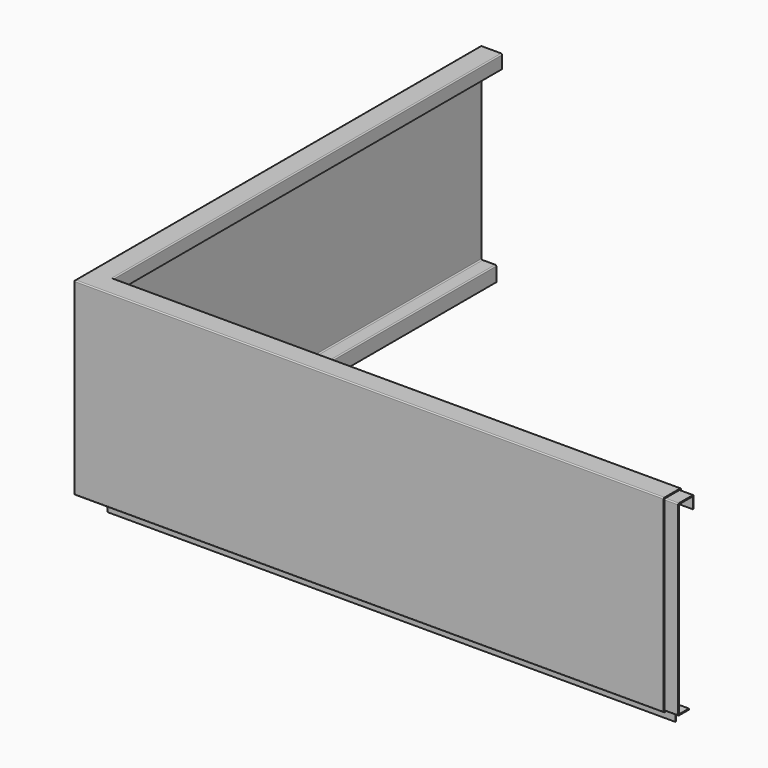
from build123d import *

# Parameters (mm, degrees)
F1_DEPTH       = 1051
F1_DEPTH_BACK  = 0.5
F3_DEPTH       = 900
F4_W           = 40
F4_H           = 40
F5_DEPTH       = 2
F7_DEPTH       = 346
F9_DEPTH       = 2
F14_D          = 5
F14_ON_F12_D   = 5
F16_DEPTH      = 25
F16_DEPTH_BACK = 25
F17_T1_DEPTH   = 50
F17_T3_DEPTH   = 1051.5
F17_T5_DEPTH   = 900
F17_T7_DEPTH   = 1069.0024143135
F17_T9_DEPTH   = 938
F17_T11_DEPTH  = 1031.5024143135
F17_T16_DEPTH  = 943.0024143135
F17_T21_DEPTH  = 1074.004828627
F17_T23_DEPTH  = 1056.0024143135
F17_T25_DEPTH  = 30.0024143135
F17_T27_DEPTH  = 1101.004828627
F17_T29_DEPTH  = 950.004828627
F17_T31_DEPTH  = 905.0024143135
F17_T33_DEPTH  = 910.004828627
F17_T38_DEPTH  = 1061.504828627
F17_T44_DEPTH  = 905.0024143135
F17_T49_DEPTH  = 1056.0024143135


# Not quite as in the source:
# - a fillet or chamfer that OpenCascade refuses, or shapes differently, is made with other operations: its cross-section is extruded or revolved along the edge and cut away or added


with BuildPart() as f1:
    # F0 (on Right) → F1 (new body, two sides)
    with BuildSketch(Plane.YZ) as f1_sk:
        Polygon((-40, 0), (-40, -350), (-13, -350), (-13, -376), (-11, -376), (-11, -348), (-38, -348), (-38, -2), (-2, -2), (-2, -25), (0, -25), (0, 0), align=None)
    extrude(amount=F1_DEPTH)
    extrude(f1_sk.sketch, amount=-F1_DEPTH_BACK)

    # F2 (on Front) → F3 (join)
    with BuildSketch(Plane.XZ):
        Polygon((-40, 0), (-40, -350), (-13, -350), (-13, -376), (-11, -376), (-11, -348), (-38, -348), (-38, -2), (-2, -2), (-2, -25), (0, -25), (0, 0), align=None)
    extrude(amount=-F3_DEPTH)

    # F4 (on Top) → F5 (join)
    with BuildSketch(Plane.XY):
        with Locations((-20, -20)):
            Rectangle(F4_W, F4_H)
    extrude(amount=-F5_DEPTH)

    # F6 (on face) → F7 (join)
    with BuildSketch(Plane(origin=(0, 0, -2), x_dir=(1, 0, 0), z_dir=(0, 0, -1))):
        Polygon((-40, 40), (-40, 0), (-38, 0), (-38, 38), (-0.5, 38), (-0.5, 40), align=None)
    extrude(amount=F7_DEPTH)

    # F8 (on face) → F9 (join)
    with BuildSketch(Plane(origin=(0, 0, -348), x_dir=(1, 0, 0), z_dir=(0, 0, -1))):
        Polygon((-40, 40), (-40, 0), (-11, 0), (-38, 38), (-0.5, 11), (0, 40), align=None)
    extrude(amount=F9_DEPTH)

    # F10: union 

    # F11: union 

    # F14 (through all)
    with Locations(Plane(origin=(-13, 0, 0), x_dir=(0, -1, 0), z_dir=(-1, 0, 0))):
        with Locations((-450, -363)):
            Hole(F14_D / 2)

    # F14 on F12 (through all)
    with Locations(Plane.XZ.offset(13)):
        with Locations((525.25, -363)):
            Hole(F14_ON_F12_D / 2)

    # F15 (on face) → F16 (join, two sides)
    with BuildSketch(Plane.YZ.offset(1051)) as f16_sk:
        Polygon((-13, -346), (-36, -346), (-36, -4), (-4, -4), (-4, -25), (-2, -25), (-2, -2), (-38, -2), (-38, -348), (-13, -348), align=None)
    extrude(amount=F16_DEPTH)
    extrude(f16_sk.sketch, amount=-F16_DEPTH_BACK)

    # F17: fillet of radius 2 on 21 edges, made by hand

    # F17_s2 → F17_t1 (join)
    with BuildSketch(Plane.YZ.offset(1026)):
        with BuildLine():
            ThreePointArc((-33.9990343146, -346.0004), (-35.4142135624, -345.4142135624), (-36.0004, -343.9990343146))
            Line((-36.0004, -343.9990343146), (-36.2005365685, -343.9990343146))
            ThreePointArc((-36.2005365685, -343.9990343146), (-36.2001365685, -344.9995171573), (-36.2001365685, -346))
            Line((-36.2001365685, -346), (-36, -346.2001365685))
            ThreePointArc((-36, -346.2001365685), (-34.9995171573, -346.2001365685), (-33.9990343146, -346.2005365685))
            Line((-33.9990343146, -346.2005365685), (-33.9990343146, -346.0004))
        make_face()
        with BuildLine():
            ThreePointArc((-6.0009656854, -3.9996), (-4.5857864376, -4.5857864376), (-3.9996, -6.0009656854))
            Line((-3.9996, -6.0009656854), (-3.7994634315, -6.0009656854))
            ThreePointArc((-3.7994634315, -6.0009656854), (-3.7998634315, -5.0004828427), (-3.7998634315, -4))
            Line((-3.7998634315, -4), (-4, -3.7998634315))
            ThreePointArc((-4, -3.7998634315), (-5.0004828427, -3.7998634315), (-6.0009656854, -3.7994634315))
            Line((-6.0009656854, -3.7994634315), (-6.0009656854, -3.9996))
        make_face()
    extrude(amount=F17_T1_DEPTH)

    # F17_s4 → F17_t3 (join)
    with BuildSketch(Plane.YZ.offset(-0.5)):
        with BuildLine():
            ThreePointArc((-15.0009656854, -349.9996), (-13.5857864376, -350.5857864376), (-12.9996, -352.0009656854))
            Line((-12.9996, -352.0009656854), (-12.7994634315, -352.0009656854))
            ThreePointArc((-12.7994634315, -352.0009656854), (-12.7998634315, -351.0004828427), (-12.7998634315, -350))
            Line((-12.7998634315, -350), (-13, -349.7998634315))
            ThreePointArc((-13, -349.7998634315), (-14.0004828427, -349.7998634315), (-15.0009656854, -349.7994634315))
            Line((-15.0009656854, -349.7994634315), (-15.0009656854, -349.9996))
        make_face()
    extrude(amount=F17_T3_DEPTH)

    # F17_s6 → F17_t5 (join)
    with BuildSketch(Plane.XZ.offset(-900)):
        with BuildLine():
            ThreePointArc((-15.0009656854, -349.9996), (-13.5857864376, -350.5857864376), (-12.9996, -352.0009656854))
            Line((-12.9996, -352.0009656854), (-12.7994634315, -352.0009656854))
            ThreePointArc((-12.7994634315, -352.0009656854), (-12.7998634315, -351.0004828427), (-12.7998634315, -350))
            Line((-12.7998634315, -350), (-13, -349.7998634315))
            ThreePointArc((-13, -349.7998634315), (-14.0004828427, -349.7998634315), (-15.0009656854, -349.7994634315))
            Line((-15.0009656854, -349.7994634315), (-15.0009656854, -349.9996))
        make_face()
        with BuildLine():
            ThreePointArc((-4.0009656854, -1.9996), (-2.5857864376, -2.5857864376), (-1.9996, -4.0009656854))
            Line((-1.9996, -4.0009656854), (-1.7994634315, -4.0009656854))
            ThreePointArc((-1.7994634315, -4.0009656854), (-1.7998634315, -3.0004828427), (-1.7998634315, -2))
            Line((-1.7998634315, -2), (-2, -1.7998634315))
            ThreePointArc((-2, -1.7998634315), (-3.0004828427, -1.7998634315), (-4.0009656854, -1.7994634315))
            Line((-4.0009656854, -1.7994634315), (-4.0009656854, -1.9996))
        make_face()
    extrude(amount=F17_T5_DEPTH)

    # F17_s8 → F17_t7 (join)
    with BuildSketch(Plane.YZ.offset(-38)):
        with BuildLine():
            ThreePointArc((-35.9990343146, -1.9996), (-37.4142135624, -2.5857864376), (-38.0004, -4.0009656854))
            Line((-38.0004, -4.0009656854), (-38.2005365685, -4.0009656854))
            ThreePointArc((-38.2005365685, -4.0009656854), (-38.2001365685, -3.0004828427), (-38.2001365685, -2))
            Line((-38.2001365685, -2), (-38, -1.7998634315))
            ThreePointArc((-38, -1.7998634315), (-36.9995171573, -1.7998634315), (-35.9990343146, -1.7994634315))
            Line((-35.9990343146, -1.7994634315), (-35.9990343146, -1.9996))
        make_face()
    extrude(amount=F17_T7_DEPTH)

    # F17_s10 → F17_t9 (join)
    with BuildSketch(Plane.XZ.offset(-900)):
        with BuildLine():
            ThreePointArc((-38.0004, -4.0009656854), (-37.4142135624, -2.5857864376), (-35.9990343146, -1.9996))
            Line((-35.9990343146, -1.9996), (-35.9990343146, -1.7994634315))
            ThreePointArc((-35.9990343146, -1.7994634315), (-36.9995171573, -1.7998634315), (-38, -1.7998634315))
            Line((-38, -1.7998634315), (-38.2001365685, -2))
            ThreePointArc((-38.2001365685, -2), (-38.2001365685, -3.0004828427), (-38.2005365685, -4.0009656854))
            Line((-38.2005365685, -4.0009656854), (-38.0004, -4.0009656854))
        make_face()
    extrude(amount=F17_T9_DEPTH)

    # F17_s12 → F17_t11 (join)
    with BuildSketch(Plane.YZ.offset(-0.5)):
        with BuildLine():
            ThreePointArc((-4.0009656854, -1.9996), (-2.5857864376, -2.5857864376), (-1.9996, -4.0009656854))
            Line((-1.9996, -4.0009656854), (-1.7994634315, -4.0009656854))
            ThreePointArc((-1.7994634315, -4.0009656854), (-1.7998634315, -3.0004828427), (-1.7998634315, -2))
            Line((-1.7998634315, -2), (-2, -1.7998634315))
            ThreePointArc((-2, -1.7998634315), (-3.0004828427, -1.7998634315), (-4.0009656854, -1.7994634315))
            Line((-4.0009656854, -1.7994634315), (-4.0009656854, -1.9996))
        make_face()
    extrude(amount=F17_T11_DEPTH)


with BuildPart() as f17_tool14:
    # F17_s15 → F17_t16 (new body)
    with BuildSketch(Plane.XZ.offset(-900)):
        with BuildLine():
            ThreePointArc((-35.9990343146, -348.0004), (-37.4142135624, -347.4142135624), (-38.0004, -345.9990343146))
            Line((-38.0004, -345.9990343146), (-38.2005365685, -345.9990343146))
            ThreePointArc((-38.2005365685, -345.9990343146), (-38.2001365685, -346.9995171573), (-38.2001365685, -348))
            Line((-38.2001365685, -348), (-38, -348.2001365685))
            ThreePointArc((-38, -348.2001365685), (-36.9995171573, -348.2001365685), (-35.9990343146, -348.2005365685))
            Line((-35.9990343146, -348.2005365685), (-35.9990343146, -348.0004))
        make_face()
    extrude(amount=F17_T16_DEPTH)

    split(bisect_by=Plane(origin=(-7.3097100782, 5.1937413714, 0), x_dir=(0, 0, 1), z_dir=(-0.8151804083, 0.5792071322, 0)), keep=Keep.TOP)


with BuildPart() as f1_1:
    add(f1.part)

    # F17_t13: union F17_tool14
    add(f17_tool14.part)


with BuildPart() as f17_tool19:
    # F17_s20 → F17_t21 (new body)
    with BuildSketch(Plane.YZ.offset(-43.0024143135)):
        with BuildLine():
            ThreePointArc((-35.9990343146, -348.0004), (-37.4142135624, -347.4142135624), (-38.0004, -345.9990343146))
            Line((-38.0004, -345.9990343146), (-38.2005365685, -345.9990343146))
            ThreePointArc((-38.2005365685, -345.9990343146), (-38.2001365685, -346.9995171573), (-38.2001365685, -348))
            Line((-38.2001365685, -348), (-38, -348.2001365685))
            ThreePointArc((-38, -348.2001365685), (-36.9995171573, -348.2001365685), (-35.9990343146, -348.2005365685))
            Line((-35.9990343146, -348.2005365685), (-35.9990343146, -348.0004))
        make_face()
    extrude(amount=F17_T21_DEPTH)

    split(bisect_by=Plane(origin=(5.0453108535, -7.0073761855, 0), x_dir=(0, 0, 1), z_dir=(0.5843047258, -0.8115343415, 0)), keep=Keep.TOP)


with BuildPart() as f1_2:
    add(f1_1.part)

    # F17_t18: union F17_tool19
    add(f17_tool19.part)

    # F17_s24 → F17_t23 (cut)
    with BuildSketch(Plane.YZ):
        with BuildLine():
            ThreePointArc((0.0004, -2.0009656854), (-0.5857864376, -0.5857864376), (-2.0009656854, 0.0004))
            Line((-2.0009656854, 0.0004), (-2.0009656854, 0.2005365685))
            ThreePointArc((-2.0009656854, 0.2005365685), (-1.0004828427, 0.2001365685), (0, 0.2001365685))
            Line((0, 0.2001365685), (0.2001365685, 0))
            ThreePointArc((0.2001365685, 0), (0.2001365685, -1.0004828427), (0.2005365685, -2.0009656854))
            Line((0.2005365685, -2.0009656854), (0.0004, -2.0009656854))
        make_face()
    extrude(amount=F17_T23_DEPTH, mode=Mode.SUBTRACT)

    # F17_s26 → F17_t25 (cut)
    with BuildSketch(Plane.YZ.offset(1051)):
        with BuildLine():
            ThreePointArc((-1.9996, -4.0009656854), (-2.5857864376, -2.5857864376), (-4.0009656854, -1.9996))
            Line((-4.0009656854, -1.9996), (-4.0009656854, -1.7994634315))
            ThreePointArc((-4.0009656854, -1.7994634315), (-3.0004828427, -1.7998634315), (-2, -1.7998634315))
            Line((-2, -1.7998634315), (-1.7998634315, -2))
            ThreePointArc((-1.7998634315, -2), (-1.7998634315, -3.0004828427), (-1.7994634315, -4.0009656854))
            Line((-1.7994634315, -4.0009656854), (-1.9996, -4.0009656854))
        make_face()
        with BuildLine():
            ThreePointArc((-35.9990343146, -1.9996), (-37.4142135624, -2.5857864376), (-38.0004, -4.0009656854))
            Line((-38.0004, -4.0009656854), (-38.2005365685, -4.0009656854))
            ThreePointArc((-38.2005365685, -4.0009656854), (-38.2001365685, -3.0004828427), (-38.2001365685, -2))
            Line((-38.2001365685, -2), (-38, -1.7998634315))
            ThreePointArc((-38, -1.7998634315), (-36.9995171573, -1.7998634315), (-35.9990343146, -1.7994634315))
            Line((-35.9990343146, -1.7994634315), (-35.9990343146, -1.9996))
        make_face()
        with BuildLine():
            ThreePointArc((-38.0004, -345.9990343146), (-37.4142135624, -347.4142135624), (-35.9990343146, -348.0004))
            Line((-35.9990343146, -348.0004), (-35.9990343146, -348.2005365685))
            ThreePointArc((-35.9990343146, -348.2005365685), (-36.9995171573, -348.2001365685), (-38, -348.2001365685))
            Line((-38, -348.2001365685), (-38.2001365685, -348))
            ThreePointArc((-38.2001365685, -348), (-38.2001365685, -346.9995171573), (-38.2005365685, -345.9990343146))
            Line((-38.2005365685, -345.9990343146), (-38.0004, -345.9990343146))
        make_face()
    extrude(amount=F17_T25_DEPTH, mode=Mode.SUBTRACT)

    # F17_s28 → F17_t27 (cut)
    with BuildSketch(Plane.YZ.offset(-45.0024143135)):
        with BuildLine():
            ThreePointArc((-40.0004, -2.0009656854), (-39.4142135624, -0.5857864376), (-37.9990343146, 0.0004))
            Line((-37.9990343146, 0.0004), (-37.9990343146, 0.2005365685))
            ThreePointArc((-37.9990343146, 0.2005365685), (-38.9995171573, 0.2001365685), (-40, 0.2001365685))
            Line((-40, 0.2001365685), (-40.2001365685, 0))
            ThreePointArc((-40.2001365685, 0), (-40.2001365685, -1.0004828427), (-40.2005365685, -2.0009656854))
            Line((-40.2005365685, -2.0009656854), (-40.0004, -2.0009656854))
        make_face()
        with BuildLine():
            ThreePointArc((-40.0004, -347.9990343146), (-39.4142135624, -349.4142135624), (-37.9990343146, -350.0004))
            Line((-37.9990343146, -350.0004), (-37.9990343146, -350.2005365685))
            ThreePointArc((-37.9990343146, -350.2005365685), (-38.9995171573, -350.2001365685), (-40, -350.2001365685))
            Line((-40, -350.2001365685), (-40.2001365685, -350))
            ThreePointArc((-40.2001365685, -350), (-40.2001365685, -348.9995171573), (-40.2005365685, -347.9990343146))
            Line((-40.2005365685, -347.9990343146), (-40.0004, -347.9990343146))
        make_face()
    extrude(amount=F17_T27_DEPTH, mode=Mode.SUBTRACT)

    # F17_s30 → F17_t29 (cut)
    with BuildSketch(Plane.XZ.offset(-905.0024143135)):
        with BuildLine():
            ThreePointArc((-40.0004, -2.0009656854), (-39.4142135624, -0.5857864376), (-37.9990343146, 0.0004))
            Line((-37.9990343146, 0.0004), (-37.9990343146, 0.2005365685))
            ThreePointArc((-37.9990343146, 0.2005365685), (-38.9995171573, 0.2001365685), (-40, 0.2001365685))
            Line((-40, 0.2001365685), (-40.2001365685, 0))
            ThreePointArc((-40.2001365685, 0), (-40.2001365685, -1.0004828427), (-40.2005365685, -2.0009656854))
            Line((-40.2005365685, -2.0009656854), (-40.0004, -2.0009656854))
        make_face()
        with BuildLine():
            ThreePointArc((-40.0004, -347.9990343146), (-39.4142135624, -349.4142135624), (-37.9990343146, -350.0004))
            Line((-37.9990343146, -350.0004), (-37.9990343146, -350.2005365685))
            ThreePointArc((-37.9990343146, -350.2005365685), (-38.9995171573, -350.2001365685), (-40, -350.2001365685))
            Line((-40, -350.2001365685), (-40.2001365685, -350))
            ThreePointArc((-40.2001365685, -350), (-40.2001365685, -348.9995171573), (-40.2005365685, -347.9990343146))
            Line((-40.2005365685, -347.9990343146), (-40.0004, -347.9990343146))
        make_face()
    extrude(amount=F17_T29_DEPTH, mode=Mode.SUBTRACT)

    # F17_s32 → F17_t31 (cut)
    with BuildSketch(Plane.XZ.offset(-905.0024143135)):
        with BuildLine():
            ThreePointArc((0.0004, -2.0009656854), (-0.5857864376, -0.5857864376), (-2.0009656854, 0.0004))
            Line((-2.0009656854, 0.0004), (-2.0009656854, 0.2005365685))
            ThreePointArc((-2.0009656854, 0.2005365685), (-1.0004828427, 0.2001365685), (0, 0.2001365685))
            Line((0, 0.2001365685), (0.2001365685, 0))
            ThreePointArc((0.2001365685, 0), (0.2001365685, -1.0004828427), (0.2005365685, -2.0009656854))
            Line((0.2005365685, -2.0009656854), (0.0004, -2.0009656854))
        make_face()
    extrude(amount=F17_T31_DEPTH, mode=Mode.SUBTRACT)

    # F17_s34 → F17_t33 (cut)
    with BuildSketch(Plane.XZ.offset(-905.0024143135)):
        with BuildLine():
            ThreePointArc((-13.0009656854, -347.9996), (-11.5857864376, -348.5857864376), (-10.9996, -350.0009656854))
            Line((-10.9996, -350.0009656854), (-10.7994634315, -350.0009656854))
            ThreePointArc((-10.7994634315, -350.0009656854), (-10.7998634315, -349.0004828427), (-10.7998634315, -348))
            Line((-10.7998634315, -348), (-11, -347.7998634315))
            ThreePointArc((-11, -347.7998634315), (-12.0004828427, -347.7998634315), (-13.0009656854, -347.7994634315))
            Line((-13.0009656854, -347.7994634315), (-13.0009656854, -347.9996))
        make_face()
    extrude(amount=F17_T33_DEPTH, mode=Mode.SUBTRACT)


with BuildPart() as f17_tool36:
    # F17_s37 → F17_t38 (new body)
    with BuildSketch(Plane.YZ.offset(-5.5024143135)):
        with BuildLine():
            ThreePointArc((-13.0009656854, -347.9996), (-11.5857864376, -348.5857864376), (-10.9996, -350.0009656854))
            Line((-10.9996, -350.0009656854), (-10.7994634315, -350.0009656854))
            ThreePointArc((-10.7994634315, -350.0009656854), (-10.7998634315, -349.0004828427), (-10.7998634315, -348))
            Line((-10.7998634315, -348), (-11, -347.7998634315))
            ThreePointArc((-11, -347.7998634315), (-12.0004828427, -347.7998634315), (-13.0009656854, -347.7994634315))
            Line((-13.0009656854, -347.7994634315), (-13.0009656854, -347.9996))
        make_face()
    extrude(amount=F17_T38_DEPTH)

    split(bisect_by=Plane.XZ.offset(13), keep=Keep.BOTTOM)


with BuildPart() as f1_3:
    add(f1_2.part)

    # F17_t35: cut F17_tool36
    add(f17_tool36.part, mode=Mode.SUBTRACT)


with BuildPart() as f17_tool42:
    # F17_s43 → F17_t44 (new body)
    with BuildSketch(Plane.XZ.offset(5.0024143135)):
        with BuildLine():
            ThreePointArc((0.0004, -2.0009656854), (-0.5857864376, -0.5857864376), (-2.0009656854, 0.0004))
            Line((-2.0009656854, 0.0004), (-2.0009656854, 0.2005365685))
            ThreePointArc((-2.0009656854, 0.2005365685), (-1.0004828427, 0.2001365685), (0, 0.2001365685))
            Line((0, 0.2001365685), (0.2001365685, 0))
            ThreePointArc((0.2001365685, 0), (0.2001365685, -1.0004828427), (0.2005365685, -2.0009656854))
            Line((0.2005365685, -2.0009656854), (0.0004, -2.0009656854))
        make_face()
    extrude(amount=-F17_T44_DEPTH)

    split(bisect_by=Plane.XZ, keep=Keep.TOP)

    split(bisect_by=Plane.XY.offset(-2), keep=Keep.TOP)


with BuildPart() as f17_tool47:
    # F17_s48 → F17_t49 (new body)
    with BuildSketch(Plane.YZ.offset(1051)):
        with BuildLine():
            ThreePointArc((0.0004, -2.0009656854), (-0.5857864376, -0.5857864376), (-2.0009656854, 0.0004))
            Line((-2.0009656854, 0.0004), (-2.0009656854, 0.2005365685))
            ThreePointArc((-2.0009656854, 0.2005365685), (-1.0004828427, 0.2001365685), (0, 0.2001365685))
            Line((0, 0.2001365685), (0.2001365685, 0))
            ThreePointArc((0.2001365685, 0), (0.2001365685, -1.0004828427), (0.2005365685, -2.0009656854))
            Line((0.2005365685, -2.0009656854), (0.0004, -2.0009656854))
        make_face()
    extrude(amount=-F17_T49_DEPTH)

    split(bisect_by=Plane.YZ, keep=Keep.BOTTOM)

    split(bisect_by=Plane.XY.offset(-2), keep=Keep.TOP)


with BuildPart() as f17_tool42_1:
    add(f17_tool42.part)

    # F17_t52: intersect F17_tool47
    add(f17_tool47.part, mode=Mode.INTERSECT)


with BuildPart() as f1_4:
    add(f1_3.part)

    # F17_t40: cut F17_tool42
    add(f17_tool42_1.part, mode=Mode.SUBTRACT)


solid = f1_4.part
